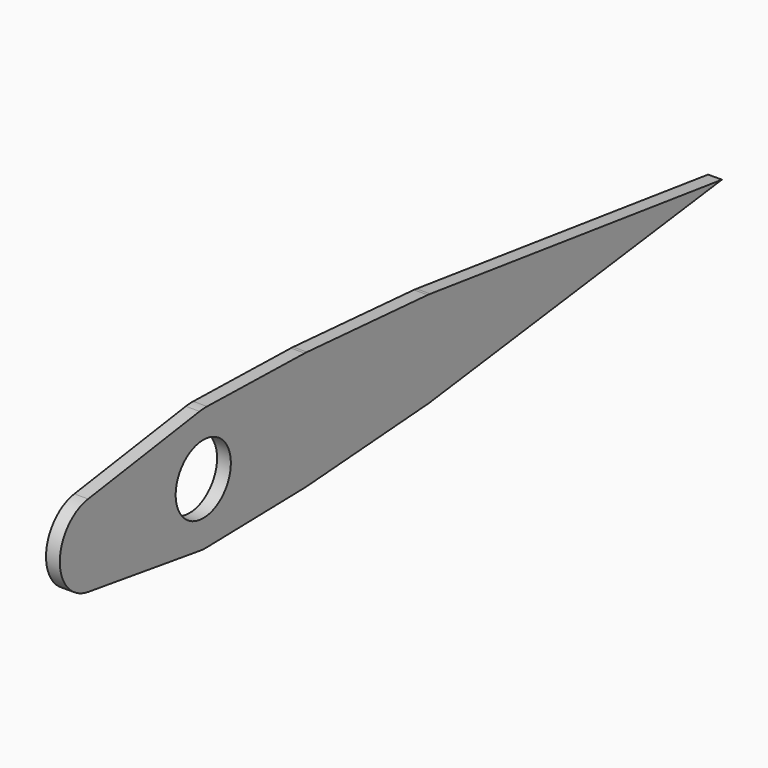
from build123d import *

# Parameters (mm, degrees)
F0_R        = 12.5
F1_DEPTH    = 2.5
F2_T1_DEPTH = 13.4446230753
F2_T3_DEPTH = 7.5224052146
F2_T5_DEPTH = 7.8412582898


# Not quite as in the source:
# - a fillet or chamfer that OpenCascade refuses, or shapes differently, is made with other operations: its cross-section is extruded or revolved along the edge and cut away or added


with BuildPart() as f1:
    # F0 (on Right) → F1 (new body, symmetric)
    with BuildSketch(Plane.YZ):
        with BuildLine():
            Line((102.2685185185, -17.3523434651), (235, 0))
            Line((235, 0), (102.2685185185, 17.3523434651))
            Line((102.2685185185, 17.3523434651), (46.4815775576, 21.4424473282))
            Line((46.4815775576, 21.4424473282), (0, 22.5))
            Line((0, 22.5), (-52.1784368395, 14.8409707545))
            ThreePointArc((-52.1784368395, 14.8409707545), (-65, 0), (-52.1784368395, -14.8409707545))
            Line((-52.1784368395, -14.8409707545), (0, -22.5))
            Line((0, -22.5), (46.4815775576, -21.4424473282))
            Line((46.4815775576, -21.4424473282), (102.2685185185, -17.3523434651))
        make_face()
        Circle(F0_R, mode=Mode.SUBTRACT)
    extrude(amount=F1_DEPTH, both=True)

    # F2: fillet of radius 20 on 4 edges, made by hand

    # F2_s2 → F2_t1 (cut)
    with BuildSketch(Plane.YZ.offset(-6.7223115376)):
        with BuildLine():
            ThreePointArc((-1.6710187212, 22.25471896), (0.0043749886, 22.428949593), (1.6884876427, 22.4615833904))
            Line((1.6884876427, 22.4615833904), (0, 22.5))
            Line((0, 22.5), (-1.6710187212, 22.25471896))
        make_face()
        with BuildLine():
            ThreePointArc((1.6884876427, -22.4615833904), (0.0043749886, -22.428949593), (-1.6710187212, -22.25471896))
            Line((-1.6710187212, -22.25471896), (0, -22.5))
            Line((0, -22.5), (1.6884876427, -22.4615833904))
        make_face()
    extrude(amount=F2_T1_DEPTH, mode=Mode.SUBTRACT)

    # F2_s4 → F2_t3 (cut)
    with BuildSketch(Plane.YZ.offset(-3.7612026073)):
        with BuildLine():
            ThreePointArc((45.9772270381, 21.4539223527), (46.4812725326, 21.4360931288), (46.9847081711, 21.4055595471))
            Line((46.9847081711, 21.4055595471), (46.4815775576, 21.4424473282))
            Line((46.4815775576, 21.4424473282), (45.9772270381, 21.4539223527))
        make_face()
    extrude(amount=F2_T3_DEPTH, mode=Mode.SUBTRACT)

    # F2_s6 → F2_t5 (cut)
    with BuildSketch(Plane.YZ.offset(-3.9206291449)):
        with BuildLine():
            ThreePointArc((101.7017879955, 17.3938941697), (102.267699979, 17.3443139587), (102.8319755439, 17.2786812132))
            Line((102.8319755439, 17.2786812132), (102.2685185185, 17.3523434651))
            Line((102.2685185185, 17.3523434651), (101.7017879955, 17.3938941697))
        make_face()
    extrude(amount=F2_T5_DEPTH, mode=Mode.SUBTRACT)


solid = f1.part
